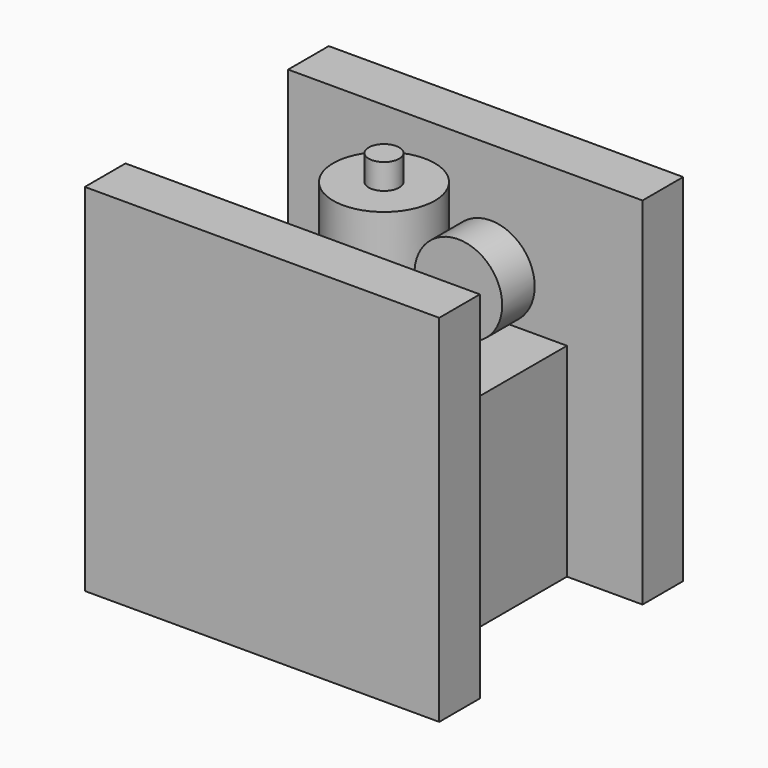
from build123d import *

# Parameters (mm, degrees)
F0_W      = 40
F0_H      = 40
F1_DEPTH  = 40
F2_R      = 3
F3_DEPTH  = 35
F5_R      = 10
F6_DEPTH  = 25
F7_R      = 8.6236634439
F8_DEPTH  = 4
F9_W      = 69.7338283062
F9_H      = 10
F10_DEPTH = 70


# Not quite as in the source:
# - the program builds the solid bodies; features that only make, move or delete a surface that nothing else refers to are left out


with BuildPart() as f1:
    # F0 (on Top) → F1 (new body)
    with BuildSketch(Plane.XY):
        Rectangle(F0_W, F0_H)
    extrude(amount=F1_DEPTH)


with BuildPart() as f3:
    # F2 (on face) → F3 (new body)
    with BuildSketch(Plane.XY.offset(40)):
        Circle(F2_R)
    extrude(amount=F3_DEPTH)

    # F5 (on offset) → F6 (join)
    with BuildSketch(Plane.XY.offset(45)):
        Circle(F5_R)
    extrude(amount=F6_DEPTH)


with BuildPart() as f8:
    # F7 (on Front) → F8 (new body, symmetric)
    with BuildSketch(Plane.XZ):
        with Locations((17.8297422826, 58.8721744716)):
            Circle(F7_R)
    extrude(amount=F8_DEPTH, both=True)


with BuildPart() as f10:
    # F9 (on Top) → F10 (new body)
    with BuildSketch(Plane.XY):
        with Locations((0, 25)):
            Rectangle(F9_W, F9_H)
    extrude(amount=F10_DEPTH)


with BuildPart() as f10b:
    # F9 (on Top) → F10, piece 2 (new body)
    with BuildSketch(Plane.XY):
        with Locations((0, -25)):
            Rectangle(F9_W, F9_H)
    extrude(amount=F10_DEPTH)


solid = Compound([f1.part, f3.part, f8.part, f10.part, f10b.part])
